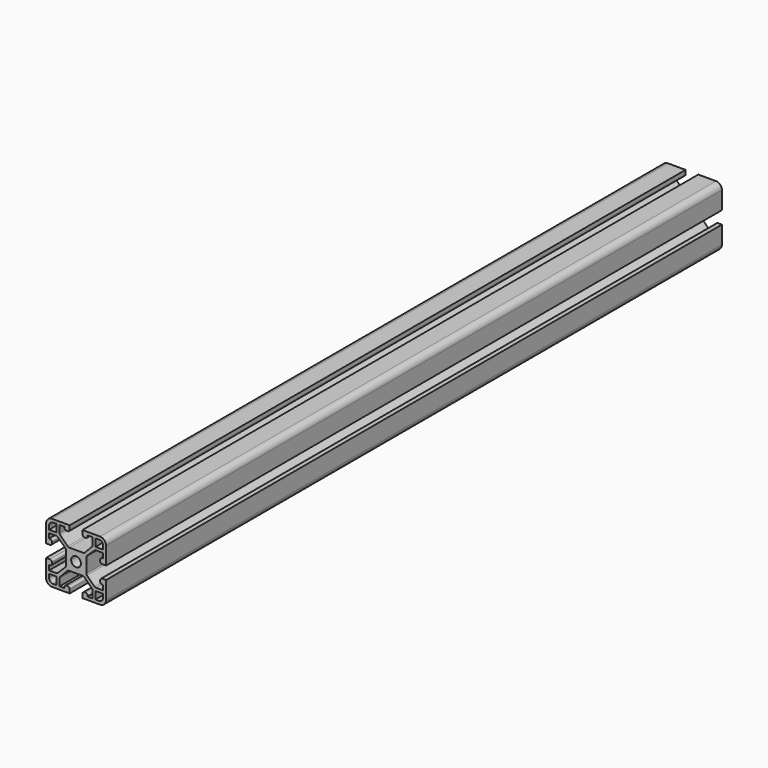
from build123d import *

# Parameters (mm, degrees)
F0_R     = 2.45
F1_DEPTH = 460
F2_DEPTH = 75


# Not quite as in the source:
# - ends of sketch curves that miss each other by under 0.0002 mm in the source are joined


with BuildPart() as f1:
    # F0 (on Front) → F1 (new body)
    with BuildSketch(Plane.XZ):
        with BuildLine():
            Line((-3.1749674082, 15), (-12, 15))
            ThreePointArc((-12, 15), (-14.1213203436, 14.1213203436), (-15, 12))
            Line((-15, 12), (-15, 3.175))
            Line((-15, 3.175), (-13.0855346263, 3.175))
            ThreePointArc((-13.0855346263, 3.175), (-12.3835980145, 3.4627605788), (-12.0856407741, 4.1604300138))
            Line((-12.0856407741, 4.1604300138), (-12.0761692778, 4.8104300138))
            ThreePointArc((-12.0761692778, 4.8104300138), (-12.3638237087, 5.5269366118), (-13.0760631299, 5.825))
            Line((-13.0760631299, 5.825), (-13.5, 5.825))
            Line((-13.5, 5.825), (-13.5, 8.225))
            Line((-13.5, 8.225), (-9.8968845016, 8.225))
            ThreePointArc((-9.8968845016, 8.225), (-9.5279915195, 8.1544718757), (-9.2111331975, 7.9528359354))
            Line((-9.2111331975, 7.9528359354), (-5.4142486959, 4.3754933338))
            ThreePointArc((-5.4142486959, 4.3754933338), (-5.1819174045, 4.0440465354), (-5.1, 3.6476573984))
            Line((-5.1, 3.6476573984), (-5.1, -3.4999243287))
            ThreePointArc((-5.1, -3.4999243287), (-5.1782354607, -3.8876744211), (-5.4007002683, -4.2147528992))
            Line((-5.4007002683, -4.2147528992), (-9.2084959767, -7.9398285705))
            ThreePointArc((-9.2084959767, -7.9398285705), (-9.5301904718, -8.1509666761), (-9.9077957084, -8.225))
            Line((-9.9077957084, -8.225), (-13.5, -8.225))
            Line((-13.5, -8.225), (-13.5, -5.825))
            Line((-13.5, -5.825), (-13.0760631299, -5.825))
            ThreePointArc((-13.0760631299, -5.825), (-12.3638237087, -5.5269366118), (-12.0761692778, -4.8104300138))
            Line((-12.0761692778, -4.8104300138), (-12.0856407741, -4.1604300138))
            ThreePointArc((-12.0856407741, -4.1604300138), (-12.3835980145, -3.4627605788), (-13.0855346263, -3.175))
            Line((-13.0855346263, -3.175), (-15, -3.175))
            Line((-15, -3.175), (-15, -12))
            ThreePointArc((-15, -12), (-14.1213203436, -14.1213203436), (-12, -15))
            Line((-12, -15), (-3.175, -15))
            Line((-3.175, -15), (-3.175, -13.0855346263))
            ThreePointArc((-3.175, -13.0855346263), (-3.4627605788, -12.3835980145), (-4.1604300138, -12.0856407741))
            Line((-4.1604300138, -12.0856407741), (-4.8104300138, -12.0761692778))
            ThreePointArc((-4.8104300138, -12.0761692778), (-5.5269366118, -12.3638237087), (-5.825, -13.0760631299))
            Line((-5.825, -13.0760631299), (-5.825, -13.5))
            Line((-5.825, -13.5), (-8.225, -13.5))
            Line((-8.225, -13.5), (-8.225, -9.8968845016))
            ThreePointArc((-8.225, -9.8968845016), (-8.1544718757, -9.5279915195), (-7.9528359354, -9.2111331975))
            Line((-7.9528359354, -9.2111331975), (-4.3754933338, -5.4142486959))
            ThreePointArc((-4.3754933338, -5.4142486959), (-4.0440465354, -5.1819174045), (-3.6476573984, -5.1))
            Line((-3.6476573984, -5.1), (3.4999243287, -5.1))
            ThreePointArc((3.4999243287, -5.1), (3.8876744211, -5.1782354607), (4.2147528992, -5.4007002683))
            Line((4.2147528992, -5.4007002683), (7.9398285705, -9.2084959767))
            ThreePointArc((7.9398285705, -9.2084959767), (8.1509666761, -9.5301904718), (8.225, -9.9077957084))
            Line((8.225, -9.9077957084), (8.225, -13.5))
            Line((8.225, -13.5), (5.825, -13.5))
            Line((5.825, -13.5), (5.825, -13.0760631299))
            ThreePointArc((5.825, -13.0760631299), (5.5269366118, -12.3638237087), (4.8104300138, -12.0761692778))
            Line((4.8104300138, -12.0761692778), (4.1604300138, -12.0856407741))
            ThreePointArc((4.1604300138, -12.0856407741), (3.4627605788, -12.3835980145), (3.175, -13.0855346263))
            Line((3.175, -13.0855346263), (3.175, -15))
            Line((3.175, -15), (12, -15))
            ThreePointArc((12, -15), (14.1213203436, -14.1213203436), (15, -12))
            Line((15, -12), (15, -3.175))
            Line((15, -3.175), (13.0855346263, -3.175))
            ThreePointArc((13.0855346263, -3.175), (12.3835980145, -3.4627605788), (12.0856407741, -4.1604300138))
            Line((12.0856407741, -4.1604300138), (12.0761692778, -4.8104300138))
            ThreePointArc((12.0761692778, -4.8104300138), (12.3638237087, -5.5269366118), (13.0760631299, -5.825))
            Line((13.0760631299, -5.825), (13.5, -5.825))
            Line((13.5, -5.825), (13.5, -8.225))
            Line((13.5, -8.225), (9.9077957084, -8.225))
            ThreePointArc((9.9077957084, -8.225), (9.5301904718, -8.1509666761), (9.2084959767, -7.9398285705))
            Line((9.2084959767, -7.9398285705), (5.4007002683, -4.2147528992))
            ThreePointArc((5.4007002683, -4.2147528992), (5.1782354607, -3.8876744211), (5.1, -3.4999243287))
            Line((5.1, -3.4999243287), (5.1, 3.6476573984))
            ThreePointArc((5.1, 3.6476573984), (5.1819174045, 4.0440465354), (5.4142486959, 4.3754933338))
            Line((5.4142486959, 4.3754933338), (9.2111331975, 7.9528359354))
            ThreePointArc((9.2111331975, 7.9528359354), (9.5279915195, 8.1544718757), (9.8968845016, 8.225))
            Line((9.8968845016, 8.225), (13.5, 8.225))
            Line((13.5, 8.225), (13.5, 5.825))
            Line((13.5, 5.825), (13.0760631299, 5.825))
            ThreePointArc((13.0760631299, 5.825), (12.3638237087, 5.5269366118), (12.0761692778, 4.8104300138))
            Line((12.0761692778, 4.8104300138), (12.0856407741, 4.1604300138))
            ThreePointArc((12.0856407741, 4.1604300138), (12.3835980145, 3.4627605788), (13.0855346263, 3.175))
            Line((13.0855346263, 3.175), (15, 3.175))
            Line((15, 3.175), (15, 12))
            ThreePointArc((15, 12), (14.1213203436, 14.1213203436), (12, 15))
            Line((12, 15), (3.1750325918, 15))
            Line((3.1750325918, 15), (3.1750325918, 13.0854824722))
            ThreePointArc((3.1750325918, 13.0854824722), (3.4627931706, 12.3835458604), (4.1604626057, 12.0855886201))
            Line((4.1604626057, 12.0855886201), (4.8104626057, 12.0761171237))
            ThreePointArc((4.8104626057, 12.0761171237), (5.5269692036, 12.3637715546), (5.8250325918, 13.0760109758))
            Line((5.8250325918, 13.0760109758), (5.8250325918, 13.4999478459))
            Line((5.8250325918, 13.4999478459), (8.2250325918, 13.4999478459))
            Line((8.2250325918, 13.4999478459), (8.2250325918, 9.8968323476))
            ThreePointArc((8.2250325918, 9.8968323476), (8.1545044675, 9.5279393654), (7.9528685272, 9.2110810434))
            Line((7.9528685272, 9.2110810434), (4.3755259256, 5.4141965418))
            ThreePointArc((4.3755259256, 5.4141965418), (4.0440791272, 5.1818652505), (3.6476899902, 5.0999478459))
            Line((3.6476899902, 5.0999478459), (-3.4998917369, 5.0999478459))
            ThreePointArc((-3.4998917369, 5.0999478459), (-3.8876418293, 5.1781833067), (-4.2147203074, 5.4006481142))
            Line((-4.2147203074, 5.4006481142), (-7.9397959787, 9.2084438226))
            ThreePointArc((-7.9397959787, 9.2084438226), (-8.1509340843, 9.5301383177), (-8.2249674082, 9.9077435543))
            Line((-8.2249674082, 9.9077435543), (-8.2249674082, 13.4999478459))
            Line((-8.2249674082, 13.4999478459), (-5.8249674082, 13.4999478459))
            Line((-5.8249674082, 13.4999478459), (-5.8249674082, 13.0760109758))
            ThreePointArc((-5.8249674082, 13.0760109758), (-5.5269040199, 12.3637715546), (-4.810397422, 12.0761171237))
            Line((-4.810397422, 12.0761171237), (-4.160397422, 12.0855886201))
            ThreePointArc((-4.160397422, 12.0855886201), (-3.462727987, 12.3835458604), (-3.1749674082, 13.0854824722))
            Line((-3.1749674082, 13.0854824722), (-3.1749674082, 15))
        make_face()
        with BuildLine():
            Line((-13.5, -11.5), (-13.5, -9.7))
            Line((-13.5, -9.7), (-9.7, -9.7))
            Line((-9.7, -9.7), (-9.7, -13.5))
            Line((-9.7, -13.5), (-11.5, -13.5))
            ThreePointArc((-11.5, -13.5), (-12.9142135624, -12.9142135624), (-13.5, -11.5))
        make_face(mode=Mode.SUBTRACT)
        with BuildLine():
            Line((9.7, -9.7), (13.5, -9.7))
            Line((13.5, -9.7), (13.5, -11.5))
            ThreePointArc((13.5, -11.5), (12.9142135624, -12.9142135624), (11.5, -13.5))
            Line((11.5, -13.5), (9.7, -13.5))
            Line((9.7, -13.5), (9.7, -9.7))
        make_face(mode=Mode.SUBTRACT)
        with BuildLine():
            ThreePointArc((-13.5, 11.5), (-12.9142135624, 12.9142135624), (-11.5, 13.5))
            Line((-11.5, 13.5), (-9.7, 13.5))
            Line((-9.7, 13.5), (-9.7, 9.7))
            Line((-9.7, 9.7), (-13.5, 9.7))
            Line((-13.5, 9.7), (-13.5, 11.5))
        make_face(mode=Mode.SUBTRACT)
        Circle(F0_R, mode=Mode.SUBTRACT)
        with BuildLine():
            Line((9.7, 13.5), (11.5, 13.5))
            ThreePointArc((11.5, 13.5), (12.9142135624, 12.9142135624), (13.5, 11.5))
            Line((13.5, 11.5), (13.5, 9.7))
            Line((13.5, 9.7), (9.7, 9.7))
            Line((9.7, 9.7), (9.7, 13.5))
        make_face(mode=Mode.SUBTRACT)
    extrude(amount=F1_DEPTH)

    # F2 (cut): a face of the model
    f2_faces = [f1.faces().sort_by_distance(p)[0] for p in [
        (5.2291627207, -460, 12.6659491494),
    ]]
    extrude(f2_faces, amount=-F2_DEPTH, mode=Mode.SUBTRACT)


solid = f1.part
